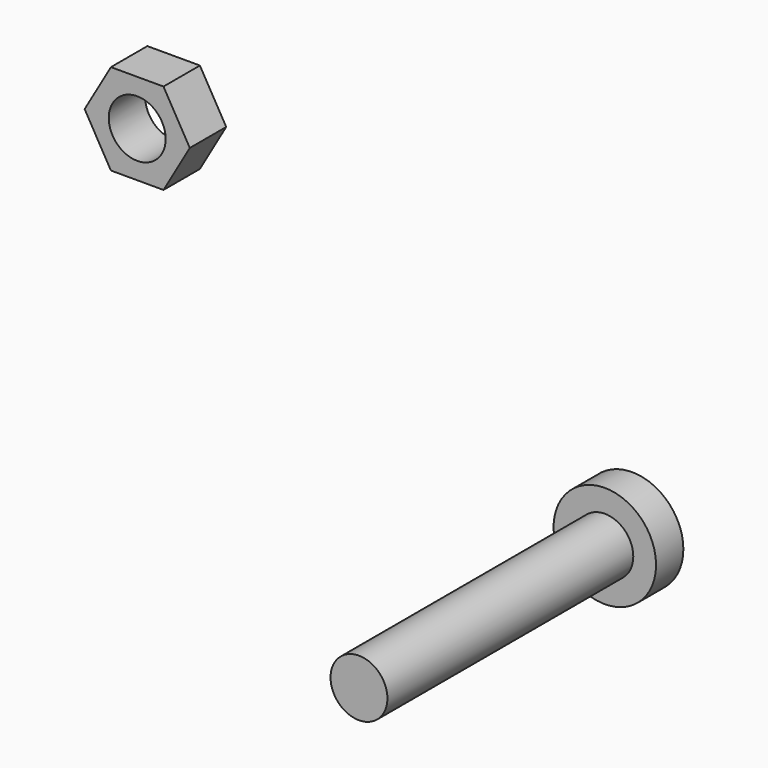
from build123d import *

# Parameters (mm, degrees)
F0_R     = 4.5
F1_DEPTH = 3
F2_R     = 2.5
F3_DEPTH = 27
F5_DEPTH = 4
F6_R     = 2.5
F7_DEPTH = 4


with BuildPart() as f1:
    # F0 (on Front) → F1 (new body)
    with BuildSketch(Plane.XZ):
        Circle(F0_R)
    extrude(amount=F1_DEPTH)

    # F2 (on face) → F3 (join)
    with BuildSketch(Plane.XZ.offset(3)):
        Circle(F2_R)
    extrude(amount=F3_DEPTH)


with BuildPart() as f5:
    # F4 (on Front) → F5 (new body)
    with BuildSketch(Plane.XZ):
        Polygon((-42.5916617033, 15.5967759937), (-37.9728595498, 15.5967759937), (-35.663458473, 19.5967759937), (-37.9728595498, 23.5967759937), (-42.5916617033, 23.5967759937), (-44.9010627801, 19.5967759937), align=None)
    extrude(amount=F5_DEPTH)

    # F6 (on face) → F7 (cut, through all)
    with BuildSketch(Plane.XZ.offset(4)):
        with Locations((-40.2822606266, 19.5967759937)):
            Circle(F6_R)
    extrude(amount=-F7_DEPTH, mode=Mode.SUBTRACT)


solid = Compound([f1.part, f5.part])
